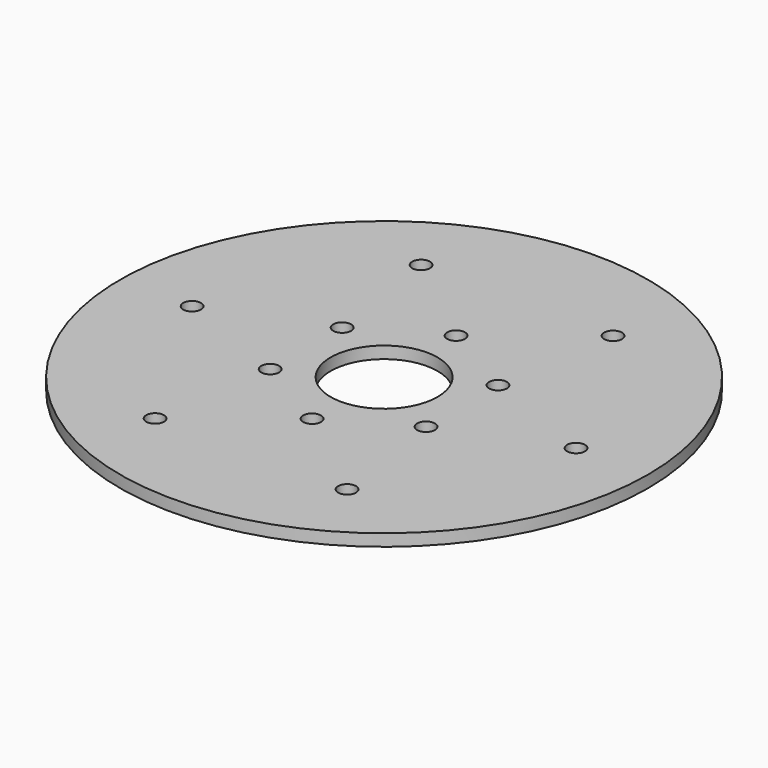
from build123d import *

# Parameters (mm, degrees)
F0_R            = 69.85
F0_R_2          = 14.1605
F1_DEPTH        = 3.175
F2_R            = 2.3622
F3_DEPTH        = 3.176
F3_COPIES_COUNT = 6


# Not quite as in the source:
# - a pattern or mirror of a feature is missing from the dataset's text; its kind, count and spacing are read off the source's solid


with BuildPart() as f1:
    # F0 (on Top) → F1 (new body)
    with BuildSketch(Plane.XY):
        Circle(F0_R)
        Circle(F0_R_2, mode=Mode.SUBTRACT)
    extrude(amount=F1_DEPTH)

    # F2 (on face) → F3 (cut, through all)
    with BuildSketch(Plane.XY.offset(3.175)):
        with Locations((0, 23.8125)):
            Circle(F2_R)
        with Locations((25.4, 43.9940905122)):
            Circle(F2_R)
    f3 = extrude(amount=-F3_DEPTH, mode=Mode.SUBTRACT)

    # F3_copies: F3 ×6 about axis
    f3_copies_axis = Axis((0, 0, 0), (0, 0, 1))
    for i in range(1, F3_COPIES_COUNT):
        add(f3.rotate(f3_copies_axis, i * 360 / F3_COPIES_COUNT), mode=Mode.SUBTRACT)


solid = f1.part
